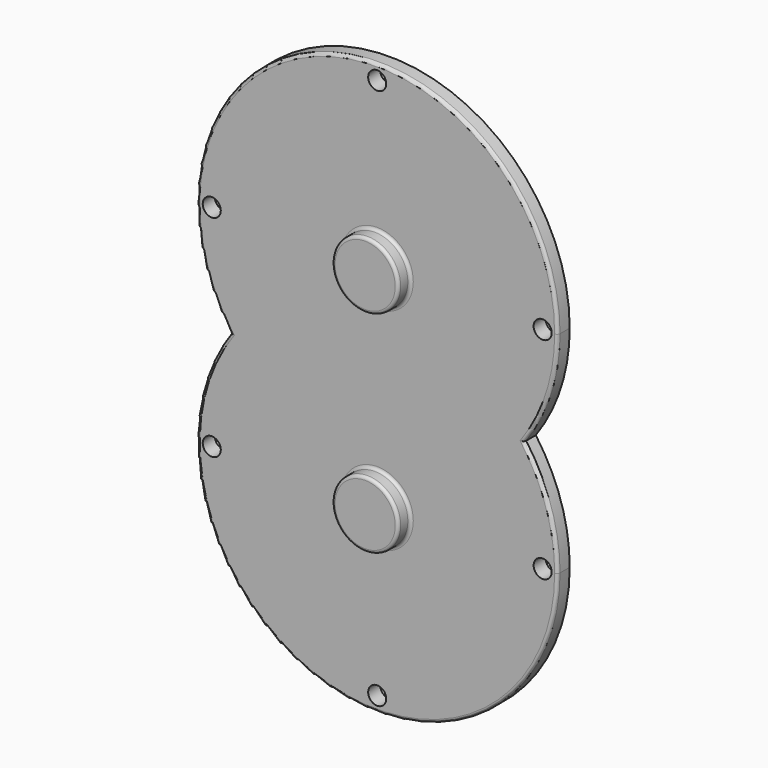
from build123d import *

# Parameters (mm, degrees)
F1_DEPTH = 5
F2_R     = 11
F3_DEPTH = 5
F4_R     = 5
F5_DEPTH = 5
F6_R     = 1
F8_D     = 6
F8_DEPTH = 20
F8_TIP   = 1.8025818571


# Not quite as in the source:
# - a pattern or mirror of a feature is missing from the dataset's text; its kind, count and spacing are read off the source's solid


with BuildPart() as f1:
    # F0 (on Front) → F1 (new body)
    with BuildSketch(Plane.XZ):
        with BuildLine():
            ThreePointArc((48.733971724, 0), (57.1140889074, 16.6157445547), (60, 35))
            ThreePointArc((60, 35), (-18.3842554453, 92.1140889074), (-48.733971724, 0))
            ThreePointArc((-48.733971724, 0), (0, 25), (48.733971724, 0))
        make_face()
        with BuildLine():
            ThreePointArc((48.733971724, 0), (0, 25), (-48.733971724, 0))
            ThreePointArc((-48.733971724, 0), (0, -25), (48.733971724, 0))
        make_face()
        with BuildLine():
            ThreePointArc((48.733971724, 0), (0, -25), (-48.733971724, 0))
            ThreePointArc((-48.733971724, 0), (-18.3842554453, -92.1140889074), (60, -35))
            ThreePointArc((60, -35), (57.1140889074, -16.6157445547), (48.733971724, 0))
        make_face()
    extrude(amount=F1_DEPTH)

    # F2 (on face) → F3 (join)
    with BuildSketch(Plane.XZ.offset(5)):
        with Locations((0, 35)):
            Circle(F2_R)
    f3 = extrude(amount=F3_DEPTH)

    # F3_copies: F3 across plane
    add(f3.mirror(Plane(origin=(0, 0, 0), x_dir=(-1, 0, 0), z_dir=(0, 0, -1))))

    # F4 (on face) → F5 (cut)
    with BuildSketch(Plane(origin=(0, 0, 0), x_dir=(-1, 0, 0), z_dir=(0, 1, 0))):
        with Locations((0, 35)):
            Circle(F4_R)
    f5 = extrude(amount=-F5_DEPTH, mode=Mode.SUBTRACT)

    # F5_copies: F5 across plane
    add(f5.mirror(Plane(origin=(0, 0, 0), x_dir=(-1, 0, 0), z_dir=(0, 0, -1))), mode=Mode.SUBTRACT)

    # F6
    f6_edges = [f1.edges().sort_by_distance(p)[0] for p in [
        (-11, -10, 35),
        (-11, -5, 35),
        (0, -5, 95),
        (0, -5, -95),
        (-11, -5, -35),
        (-11, -10, -35),
    ]]
    fillet(f6_edges, radius=F6_R)

    # F8
    with Locations(Plane.XZ.offset(5)):
        with Locations((0, 90), (-55, 35), (-55, -35), (0, -90), (55, -35), (55, 35)):
            Hole(F8_D / 2, depth=F8_DEPTH)
            with Locations((0, 0, -(F8_DEPTH + F8_TIP / 2))):  # 118° drill point
                Cone(0, F8_D / 2, F8_TIP, mode=Mode.SUBTRACT)


solid = f1.part
